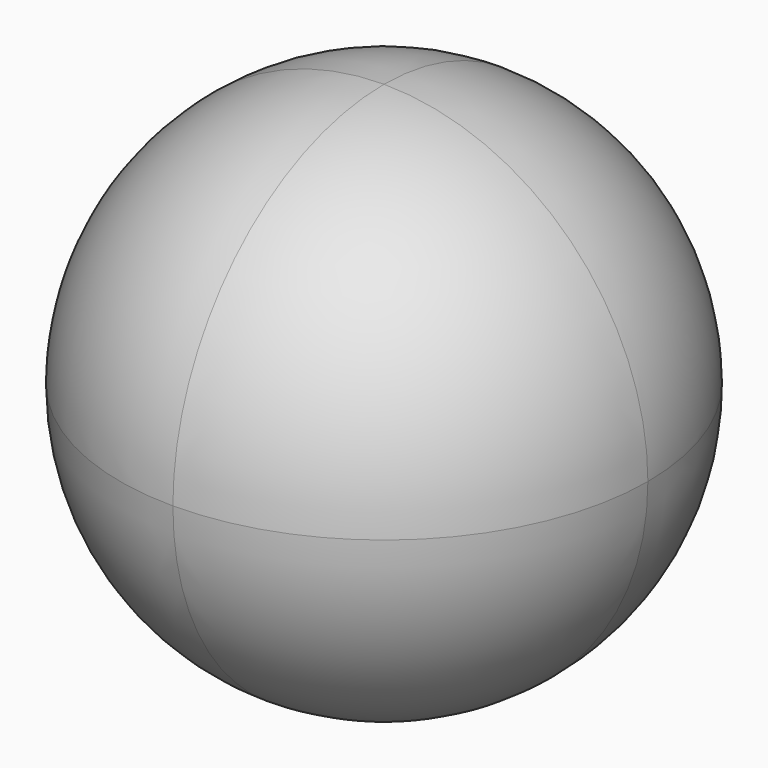
from build123d import *

# Parameters (mm, degrees)
F0_W          = 3.81
F0_H          = 3.81
F1_DEPTH      = 1.905
F1_DEPTH_BACK = 1.905
F2_R          = 1.90499


# Not quite as in the source:
# - a fillet or chamfer is up to 0.001 mm smaller than in the source, because OpenCascade refuses the exact size


with BuildPart() as f1:
    # F0 (on Front) → F1 (new body, two sides)
    with BuildSketch(Plane.XZ) as f1_sk:
        Rectangle(F0_W, F0_H)
    extrude(amount=F1_DEPTH)
    extrude(f1_sk.sketch, amount=-F1_DEPTH_BACK)

    # F2 (radius 1.905 in the source; OpenCascade refuses exactly that, so slightly less here)
    f2_edges = [f1.edges().sort_by_distance(p)[0] for p in [
        (1.905, -1.905, 0),
        (0, -1.905, 1.905),
        (-1.905, -1.905, 0),
        (0, -1.905, -1.905),
        (-1.905, 0, 1.905),
        (0, 1.905, 1.905),
        (1.905, 0, 1.905),
        (1.905, 0, -1.905),
        (1.905, 1.905, 0),
        (-1.905, 1.905, 0),
        (0, 1.905, -1.905),
        (-1.905, 0, -1.905),
    ]]
    fillet(f2_edges, radius=F2_R)


solid = f1.part
